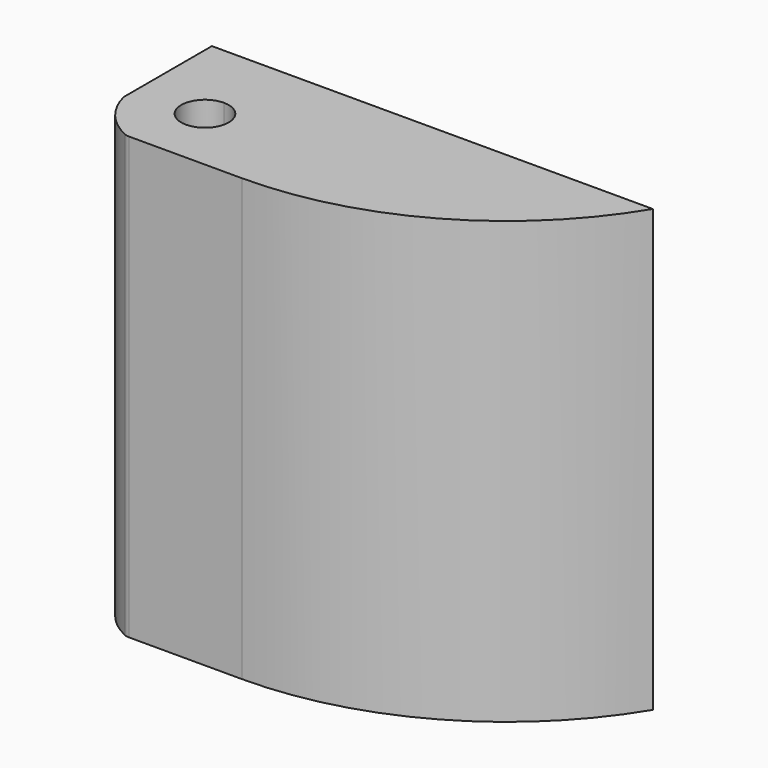
from build123d import *

# Parameters (mm, degrees)
F1_DEPTH    = 40
F2_R        = 1
F3_T1_DEPTH = 168.4279953904


# Not quite as in the source:
# - a fillet or chamfer that OpenCascade refuses, or shapes differently, is made with other operations: its cross-section is extruded or revolved along the edge and cut away or added


with BuildPart() as f1:
    # F0 (on Top) → F1 (new body)
    with BuildSketch(Plane.XY):
        with BuildLine():
            Line((0, 2.15), (0, 8.41))
            Line((0, 8.41), (-6.1, 8.41))
            Line((-6.1, 8.41), (-6.1, -1.59))
            ThreePointArc((-6.1, -1.59), (-4.7073896383, -4.2954889128), (-2.25, -6.09))
            Line((-2.25, -6.09), (0, -6.09))
            Line((0, -6.09), (0, -2.15))
            ThreePointArc((0, -2.15), (-2.15, 0), (0, 2.15))
        make_face()
        with BuildLine():
            Line((6.1, -1.59), (6.1, 8.41))
            Line((6.1, 8.41), (0, 8.41))
            Line((0, 8.41), (0, 2.15))
            ThreePointArc((0, 2.15), (1.5202795796, 1.5202795796), (2.15, 0))
            ThreePointArc((2.15, 0), (1.5202795796, -1.5202795796), (0, -2.15))
            Line((0, -2.15), (0, -6.09))
            Line((0, -6.09), (2.25, -6.09))
            ThreePointArc((2.25, -6.09), (4.7073896383, -4.2954889128), (6.1, -1.59))
        make_face()
        with BuildLine():
            Line((33.9, 8.41), (6.1, 8.41))
            Line((6.1, 8.41), (6.1, -1.59))
            ThreePointArc((6.1, -1.59), (4.7073896383, -4.2954889128), (2.25, -6.09))
            Line((2.25, -6.09), (33.9, -6.09))
            Line((33.9, -6.09), (33.9, 8.41))
        make_face()
    extrude(amount=F1_DEPTH)

    # F2
    f2_edges = [f1.edges().sort_by_distance(p)[0] for p in [
        (-2.25, -6.09, 20),
    ]]
    fillet(f2_edges, radius=F2_R)

    # F3: fillet of radius 30 on 1 edges, made by hand

    # F3_s2 → F3_t1 (cut)
    with BuildSketch(Plane.XY.offset(-64.2139976952)):
        with BuildLine():
            ThreePointArc((8.2144009219, -6.09), (22.9622821257, -2.2147009552), (33.9, 8.41))
            Line((33.9, 8.41), (33.9, -6.09))
            Line((33.9, -6.09), (8.2144009219, -6.09))
        make_face()
    extrude(amount=F3_T1_DEPTH, mode=Mode.SUBTRACT)


solid = f1.part
